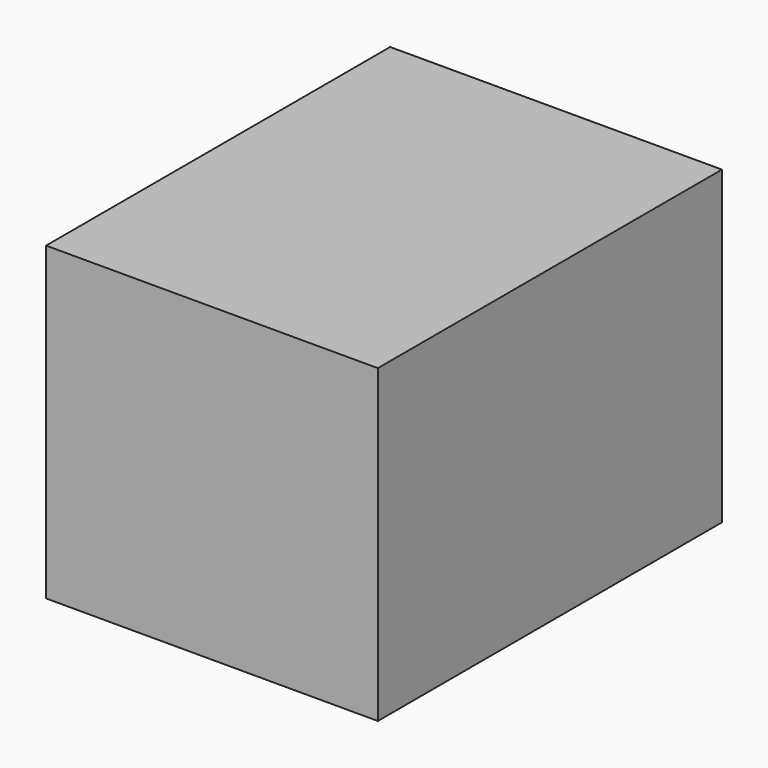
from build123d import *

# Parameters (mm, degrees)
F0_W     = 39.1885712743
F0_H     = 36.6912633181
F1_DEPTH = 50.8


# Not quite as in the source:
# - a feature names something its author has since deleted; it is built from what else it names


with BuildPart() as f1:
    # F0 (on Front) → F1 (new body)
    with BuildSketch(Plane.XZ):
        Rectangle(F0_W, F0_H)
    extrude(amount=F1_DEPTH)


solid = f1.part
